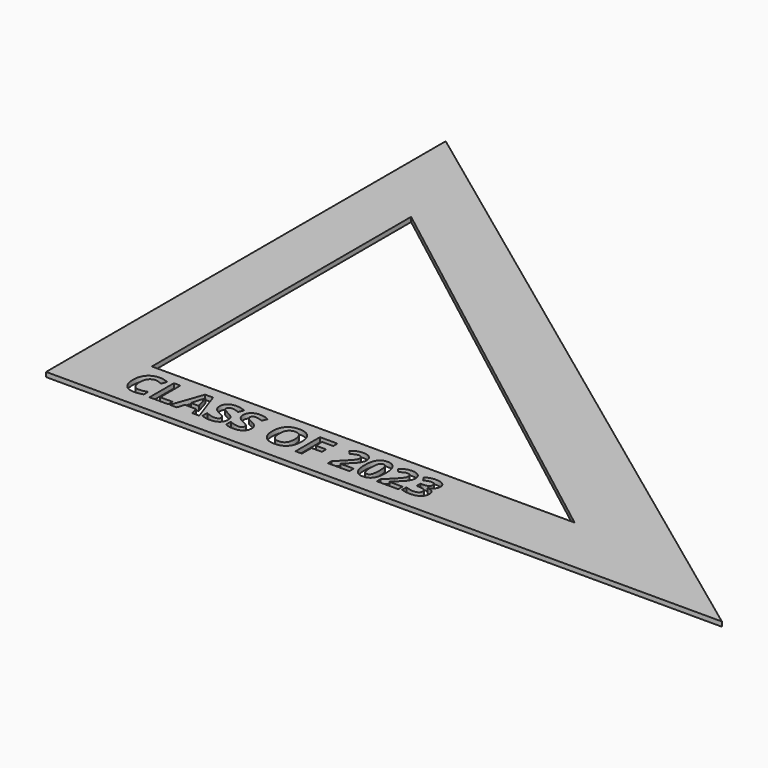
from build123d import *

# Parameters (mm, degrees)
F1_DEPTH     = 2
F2_SCALE     = 0.75
F3_TEXT_SIZE = 13.8751121122
F4_DEPTH     = 1.501


# Not quite as in the source:
# - Text() gives the source's letters only with a copy of the font that has no kerning and outlines rounded to 1/6400 em; it was checked with that copy


with BuildPart() as f1:
    # F0 (on Top) → F1 (new body)
    with BuildSketch(Plane.XY):
        Polygon((-110.3935540405, 109.5033976257), (-110.3935540405, -106.3966023743), (181.7064459595, -106.3966023743), align=None)
        Polygon((-84.9935540405, -80.9966023743), (-84.9935540405, 59.0477188125), (97.7188157638, -80.9966023743), align=None, mode=Mode.SUBTRACT)
    extrude(amount=F1_DEPTH)


with BuildPart() as f1_1:
    # F2: moved
    add(f1.part.scale(F2_SCALE))

    # F3 (on face) → F4 (cut, through all)
    with BuildSketch(Plane.XY.offset(1.5)):
        with Locations((-63.7451655304, -74.3297189474)):
            Text('CLASS OF 2023', F3_TEXT_SIZE, font='Open Sans', font_style=FontStyle.BOLD, text_align=(TextAlign.LEFT, TextAlign.BOTTOM))
    extrude(amount=-F4_DEPTH, mode=Mode.SUBTRACT)


solid = f1_1.part
